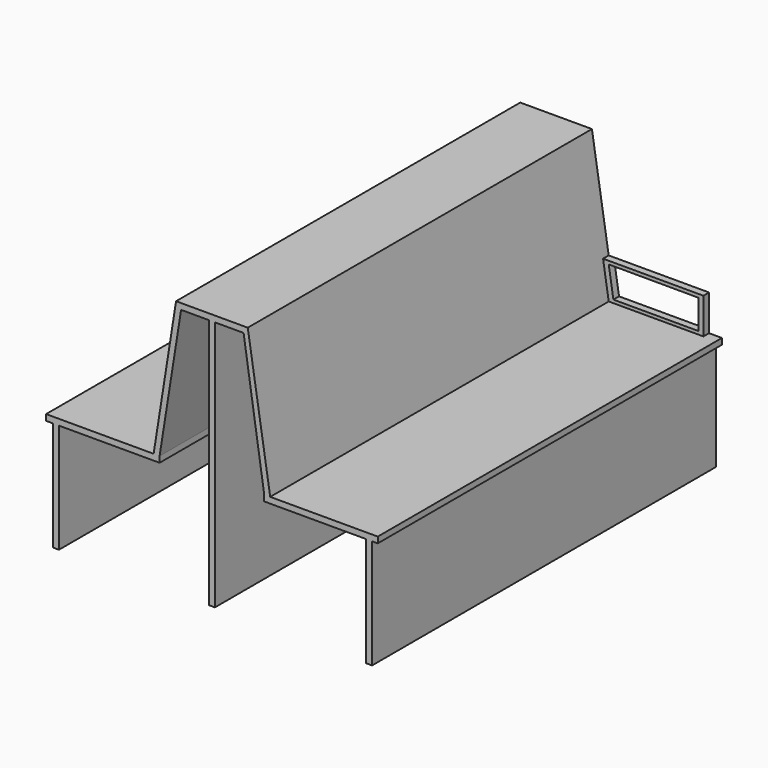
from build123d import *

# Parameters (mm, degrees)
F0_W     = 25.4
F0_H     = 464.7051875732
F0_H_2   = 1066.8
F0_H_3   = 25.4
F1_DEPTH = 1828.8
F2_DEPTH = 30


# Not quite as in the source:
# - a feature names something its author has since deleted; it is built from what else it names


with BuildPart() as f1:
    # F0 (on Front) → F1 (new body)
    with BuildSketch(Plane.XZ):
        with Locations((-415.2822112945, -802.4841870543)):
            Rectangle(F0_W, F0_H)
        with Locations((247.7624498885, -501.4367808409)):
            Rectangle(F0_W, F0_H_2)
        with Locations((915.8871110716, -802.4841870543)):
            Rectangle(F0_W, F0_H)
        with Locations((12.7, -557.4315932677)):
            Rectangle(F0_W, F0_H_3)
        Polygon((145.9203362465, 57.3632191591), (95.3624498885, 57.3632191591), (24.1377887055, -392.3315932677), (0, -544.7315932677), (25.4, -544.7315932677), (116.7394851043, 31.9632191591), (145.9203362465, 31.9632191591), align=None)
        Polygon((362.7394139767, 57.3632191591), (145.9203362465, 57.3632191591), (145.9203362465, 31.9632191591), (235.0624498885, 31.9632191591), (260.4624498885, 31.9632191591), (362.7394139767, 31.9632191591), align=None)
        Polygon((898.1071110716, -544.7315932677), (495.524899777, -544.7315932677), (470.124899777, -544.7315932677), (470.124899777, -570.1315932677), (903.1871110716, -570.1315932677), (928.5871110716, -570.1315932677), (952.7248997771, -570.1315932677), (952.724899777, -544.7315932677), align=None)
        Polygon((400.1624498885, 57.3632191591), (362.7394139767, 57.3632191591), (362.7394139767, 31.9632191591), (382.4598755032, 31.9632191591), (470.124899777, -544.7315932677), (495.524899777, -544.7315932677), (471.3871110716, -392.3315932677), align=None)
        Polygon((0, -570.1315932677), (0, -544.7315932677), (-402.5822112945, -544.7315932677), (-457.2, -544.7315932677), (-457.2, -570.1315932677), (-427.9822112945, -570.1315932677), (-402.5822112945, -570.1315932677), align=None)
    extrude(amount=F1_DEPTH)

    # F0 (on Front) → F2 (join)
    with BuildSketch(Plane.XZ):
        Polygon((0, -544.7315932677), (24.1377887055, -392.3315932677), (-402.5822112945, -392.3315932677), (-402.5822112945, -544.7315932677), align=None)
        Polygon((-382.1481764317, -406.8649113178), (0, -406.0111343861), (-19.8426051641, -531.2924127962), (-382.1481764317, -531.2924127962), align=None, mode=Mode.SUBTRACT)
        Polygon((898.1071110716, -392.3315932677), (471.3871110716, -392.3315932677), (495.524899777, -544.7315932677), (898.1071110716, -544.7315932677), align=None)
        Polygon((495.524899777, -406.0111343861), (877.6730762087, -406.8649113178), (877.6730762087, -531.2924127962), (515.3675049412, -531.2924127962), align=None, mode=Mode.SUBTRACT)
    extrude(amount=F2_DEPTH)


solid = f1.part
